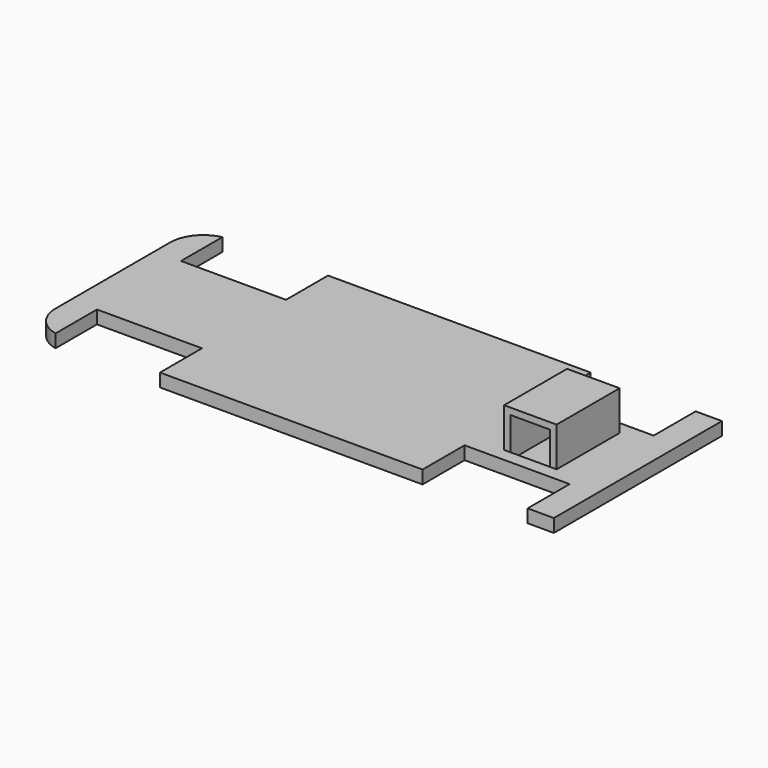
from build123d import *

# Parameters (mm, degrees)
F0_W        = 20
F0_H        = 30
F1_DEPTH    = 20
F0_W_2      = 10
F0_H_2      = 40
F0_W_3      = 40
F0_H_3      = 20
F2_DEPTH    = 5
F3_T        = 2.5
F3_T3_DEPTH = 25
F3_T5_DEPTH = 35
F3_T7_DEPTH = 10


# Not quite as in the source:
# - a shell that OpenCascade refuses in one call is made with other operations: the cavity is built on its own and cut out


with BuildPart() as f1:
    # F0 (on Top) → F1 (new body)
    with BuildSketch(Plane.XY):
        with Locations((71.046166122, 0)):
            Rectangle(F0_W, F0_H)
    extrude(amount=F1_DEPTH)

    # F0 (on Top) → F2 (join)
    with BuildSketch(Plane.XY):
        with BuildLine():
            ThreePointArc((-90, 39.709673646), (-97.1888826467, 35.2686887253), (-100, 27.3))
            Line((-100, 27.3), (-100, 20))
            Line((-100, 20), (-90, 20))
            Line((-90, 20), (-90, 39.709673646))
        make_face()
        with Locations((-95, 0)):
            Rectangle(F0_W_2, F0_H_2)
        with BuildLine():
            Line((-90, -20), (-100, -20))
            Line((-100, -20), (-100, -27.3))
            ThreePointArc((-100, -27.3), (-97.1888826467, -35.2686887253), (-90, -39.709673646))
            Line((-90, -39.709673646), (-90, -20))
        make_face()
        with Locations((-70, 0)):
            Rectangle(F0_W_3, F0_H_2)
        Polygon((-50, 40), (-50, 20), (-50, -20), (-50, -40), (50, -40), (50, -20), (50, 20), (50, 40), align=None)
        with Locations((70, 0)):
            Rectangle(F0_W_3, F0_H_2)
        with Locations((71.046166122, 0)):
            Rectangle(F0_W, F0_H, mode=Mode.SUBTRACT)
        with Locations((95, 0)):
            Rectangle(F0_W_2, F0_H_2)
        with Locations((95, -30)):
            Rectangle(F0_W_2, F0_H_3)
        with Locations((95, 30)):
            Rectangle(F0_W_2, F0_H_3)
    extrude(amount=F2_DEPTH)

    # F3: shell of thickness 2.5, made by hand


with BuildPart() as f3_core1:
    # F3_t2: copy of F1
    add(f1.part)

    # the walls: a layer under each face that stays
    f3_faces = [f3_core1.faces().sort_by_distance(p)[0] for p in [
        (71.046166122, 15, 12.5),
        (0, 0, 5),
        (61.046166122, 0, 12.5),
        (71.046166122, 0, 20),
        (81.046166122, 0, 12.5),
        (-97.1888826467, 35.2686887253, 2.5),
        (-100, 0, 2.5),
        (-97.1888826467, -35.2686887253, 2.5),
        (-90, -29.854836823, 2.5),
        (-70, -20, 2.5),
        (-50, -30, 2.5),
        (0, -40, 2.5),
        (50, -30, 2.5),
        (70, -20, 2.5),
        (90, -30, 2.5),
        (95, -40, 2.5),
        (100, 0, 2.5),
        (95, 40, 2.5),
        (90, 30, 2.5),
        (70, 20, 2.5),
        (50, 30, 2.5),
        (0, 40, 2.5),
        (-50, 30, 2.5),
        (-70, 20, 2.5),
        (-90, 29.854836823, 2.5),
        (0, 0, 0),
    ]]
    thicken(f3_faces, amount=-F3_T, mode=Mode.SUBTRACT)

    # F3_s4 → F3_t3 (cut)
    with BuildSketch(Plane.YZ.offset(58.546166122)):
        Polygon((15.025, 5.025), (12.5, 5), (12.5, 2.5), (15, 2.5), align=None)
    extrude(amount=F3_T3_DEPTH, mode=Mode.SUBTRACT)

    # F3_s6 → F3_t5 (cut)
    with BuildSketch(Plane.XZ.offset(-17.5)):
        Polygon((61.021166122, 5.025), (61.046166122, 2.5), (63.546166122, 2.5), (63.546166122, 5), align=None)
        Polygon((81.071166122, 5.025), (81.046166122, 2.5), (78.546166122, 2.5), (78.546166122, 5), align=None)
    extrude(amount=F3_T5_DEPTH, mode=Mode.SUBTRACT)

    # F3_s8 → F3_t7 (cut)
    with BuildSketch(Plane.XY.offset(-2.5)):
        Polygon((-89.975, -20.025), (-92.5, -20), (-92.5, -17.5), (-90, -17.5), align=None)
        Polygon((-50.025, -20.025), (-50, -17.5), (-47.5, -17.5), (-47.5, -20), align=None)
        Polygon((50.025, -20.025), (47.5, -20), (47.5, -17.5), (50, -17.5), align=None)
        Polygon((89.975, -20.025), (90, -17.5), (92.5, -17.5), (92.5, -20), align=None)
        Polygon((89.975, 20.025), (92.5, 20), (92.5, 17.5), (90, 17.5), align=None)
        Polygon((50.025, 20.025), (50, 17.5), (47.5, 17.5), (47.5, 20), align=None)
        Polygon((-50.025, 20.025), (-47.5, 20), (-47.5, 17.5), (-50, 17.5), align=None)
        Polygon((-89.975, 20.025), (-90, 17.5), (-92.5, 17.5), (-92.5, 20), align=None)
    extrude(amount=F3_T7_DEPTH, mode=Mode.SUBTRACT)


with BuildPart() as f1_1:
    add(f1.part)

    # what is left inside the walls is the cavity
    f3_cavity = [f3_core1.part.solids().sort_by_distance(p)[0] for p in [
        (71.046166, -5.833333, 17.475),
    ]]
    add(f3_cavity, mode=Mode.SUBTRACT)


solid = f1_1.part
